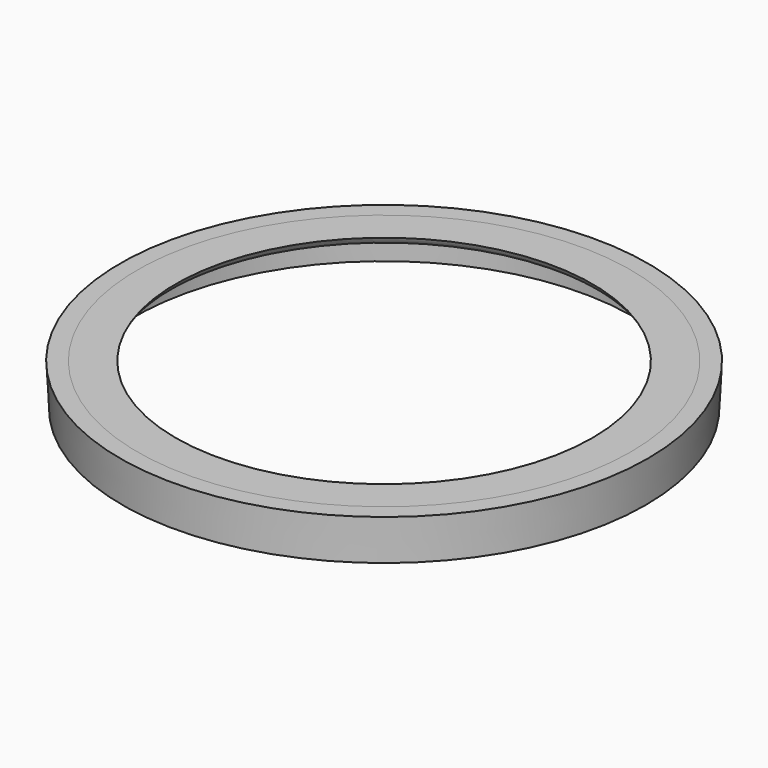
from build123d import *

# Parameters (mm, degrees)
F0_R     = 76
F0_R_2   = 71
F1_DEPTH = 12
F1_TAPER = 3
F0_R_3   = 65
F0_R_4   = 60
F2_DEPTH = 3
F6_R     = 2.99999


# Not quite as in the source:
# - a fillet or chamfer that OpenCascade refuses, or shapes differently, is made with other operations: its cross-section is extruded or revolved along the edge and cut away or added
# - a fillet or chamfer is up to 0.001 mm smaller than in the source, because OpenCascade refuses the exact size


with BuildPart() as f1:
    # F0 (on Top) → F1 (new body)
    with BuildSketch(Plane.XY):
        Circle(F0_R)
        Circle(F0_R_2, mode=Mode.SUBTRACT)
    extrude(amount=-F1_DEPTH, taper=F1_TAPER)


with BuildPart() as f2:
    # F0 (on Top) → F2 (new body)
    with BuildSketch(Plane.XY):
        Circle(F0_R_2)
        Circle(F0_R_3, mode=Mode.SUBTRACT)
        Circle(F0_R_3)
        Circle(F0_R_4, mode=Mode.SUBTRACT)
    extrude(amount=-F2_DEPTH)

    # F5: fillet of radius 5 on 1 edges, made by hand

    # F5_s1 → F5_t2 (revolve, cut)
    with BuildSketch(Plane.XZ):
        with BuildLine():
            ThreePointArc((60, 0), (61.8439629074, -2.1833001327), (64.582575695, -3))
            Line((64.582575695, -3), (60, -3))
            Line((60, -3), (60, 0))
        make_face()
    revolve(axis=Axis((0, 0, -3), (0, 0, 1)), mode=Mode.SUBTRACT)

    # F6 (radius 3 in the source; OpenCascade refuses exactly that, so slightly less here)
    f6_edges = [f2.edges().sort_by_distance(p)[0] for p in [
        (-71, 0, -3),
    ]]
    fillet(f6_edges, radius=F6_R)


solid = Compound([f1.part, f2.part])
